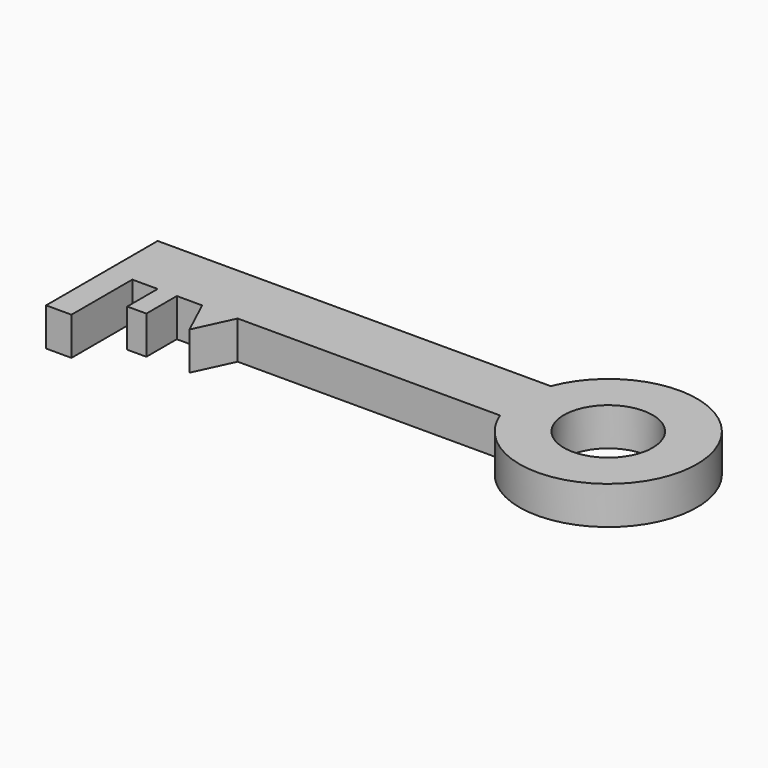
from build123d import *

# Parameters (mm, degrees)
F0_W     = 7.5505197141
F0_H     = 15
F0_W_2   = 10
F0_H_2   = 30
F0_R     = 17.5
F1_DEPTH = 15


# Not quite as in the source:
# - a feature of the source that left no trace in its solid (it failed there, or was rolled back) is left out


with BuildPart() as f1:
    # F0 (on Top) → F1 (new body)
    with BuildSketch(Plane.XY):
        Polygon((63.855322471, 51.9168977576), (-91.144677529, 51.9168977576), (-91.144677529, 26.9168977576), (-81.144677529, 26.9168977576), (-71.144677529, 26.9168977576), (-63.594157815, 26.9168977576), (-53.594157815, 26.9168977576), (-46.594157815, 26.9168977576), (-39.594157815, 26.9168977576), (63.855322471, 26.9168977576), align=None)
        Polygon((-46.594157815, 11.9168977576), (-39.594157815, 26.9168977576), (-46.594157815, 26.9168977576), (-53.594157815, 26.9168977576), align=None)
        with Locations((-67.369417672, 19.4168977576)):
            Rectangle(F0_W, F0_H)
        with Locations((-86.144677529, 11.9168977576)):
            Rectangle(F0_W_2, F0_H_2)
        with BuildLine():
            ThreePointArc((63.855322471, 26.9168977576), (131.5470645475, 39.4168977576), (63.855322471, 51.9168977576))
            Line((63.855322471, 51.9168977576), (63.855322471, 26.9168977576))
        make_face()
        with Locations((96.5470645475, 39.4168977576)):
            Circle(F0_R, mode=Mode.SUBTRACT)
    extrude(amount=F1_DEPTH)


solid = f1.part
